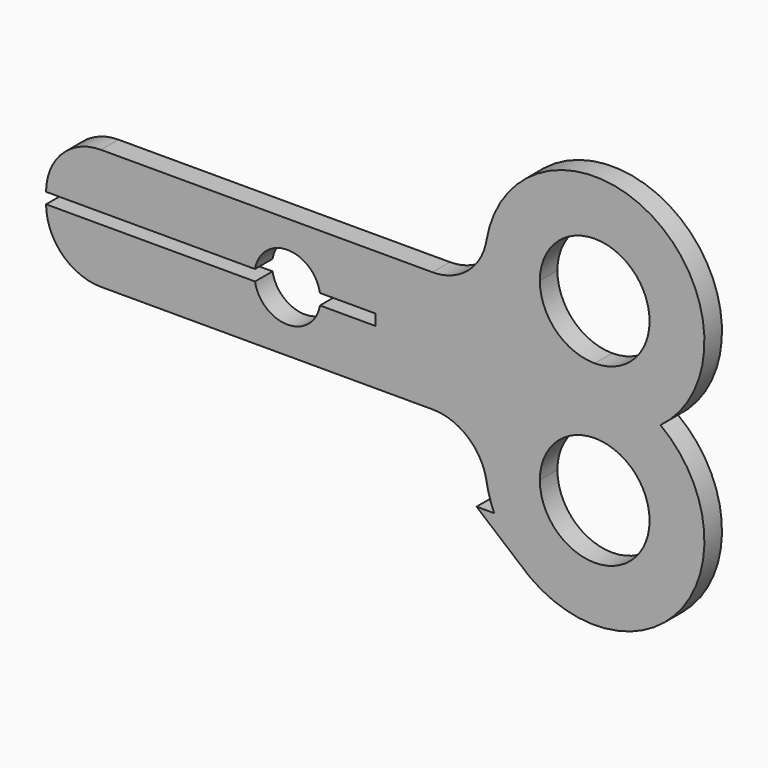
from build123d import *

# Parameters (mm, degrees)
F1_DEPTH = 2
F2_R     = 5
F4_DEPTH = 2
F6_DEPTH = 2


# Not quite as in the source:
# - a feature names something its author has since deleted; it is built from what else it names


with BuildPart() as f1:
    # F0 (on Front) → F1 (new body)
    with BuildSketch(Plane.XZ):
        with BuildLine():
            Line((0, 5.5), (0, 0))
            Line((0, 0), (40, 0))
            Line((40, 0), (40, 5.5))
            Line((40, 5.5), (25, 5.5))
            ThreePointArc((25, 5.5), (22, 2.5), (19, 5.5))
            Line((19, 5.5), (0, 5.5))
        make_face()
        with BuildLine():
            Line((40, 5.5), (40, 0))
            Line((40, 0), (40, -2.5))
            ThreePointArc((40, -2.5), (41.05572809, 1.972135955), (44, 5.5))
            Line((44, 5.5), (40, 5.5))
        make_face()
        with BuildLine():
            Line((0, 11), (0, 5.5))
            Line((0, 5.5), (19, 5.5))
            ThreePointArc((19, 5.5), (22, 8.5), (25, 5.5))
            Line((25, 5.5), (40, 5.5))
            Line((40, 5.5), (40, 11))
            Line((40, 11), (0, 11))
        make_face()
        with BuildLine():
            Line((40, 11), (40, 5.5))
            Line((40, 5.5), (44, 5.5))
            ThreePointArc((44, 5.5), (41.05572809, 9.027864045), (40, 13.5))
            Line((40, 13.5), (40, 11))
        make_face()
        with BuildLine():
            Line((45, -2.5), (40, -2.5))
            ThreePointArc((40, -2.5), (50, -12.5), (60, -2.5))
            ThreePointArc((60, -2.5), (58.94427191, 1.972135955), (56, 5.5))
            ThreePointArc((56, 5.5), (53.1622776602, 4.0131670195), (50, 3.5))
            Line((50, 3.5), (50, 2.5))
            ThreePointArc((50, 2.5), (53.5355339059, 1.0355339059), (55, -2.5))
            ThreePointArc((55, -2.5), (50, -7.5), (45, -2.5))
        make_face()
        with BuildLine():
            ThreePointArc((44, 5.5), (41.05572809, 1.972135955), (40, -2.5))
            Line((40, -2.5), (45, -2.5))
            ThreePointArc((45, -2.5), (46.4644660941, 1.0355339059), (50, 2.5))
            Line((50, 2.5), (50, 3.5))
            ThreePointArc((50, 3.5), (46.8377223398, 4.0131670195), (44, 5.5))
        make_face()
        with BuildLine():
            ThreePointArc((40, 13.5), (41.05572809, 9.027864045), (44, 5.5))
            ThreePointArc((44, 5.5), (46.8377223398, 6.9868329805), (50, 7.5))
            Line((50, 7.5), (50, 8.5))
            ThreePointArc((50, 8.5), (46.4644660941, 9.9644660941), (45, 13.5))
            Line((45, 13.5), (40, 13.5))
        make_face()
        with BuildLine():
            Line((50, 5.5), (44, 5.5))
            ThreePointArc((44, 5.5), (46.8377223398, 4.0131670195), (50, 3.5))
            Line((50, 3.5), (50, 5.5))
        make_face()
        with BuildLine():
            ThreePointArc((50, 7.5), (46.8377223398, 6.9868329805), (44, 5.5))
            Line((44, 5.5), (50, 5.5))
            Line((50, 5.5), (50, 7.5))
        make_face()
        with BuildLine():
            ThreePointArc((60, 13.5), (50, 23.5), (40, 13.5))
            Line((40, 13.5), (45, 13.5))
            ThreePointArc((45, 13.5), (50, 18.5), (55, 13.5))
            ThreePointArc((55, 13.5), (53.5355339059, 9.9644660941), (50, 8.5))
            Line((50, 8.5), (50, 7.5))
            ThreePointArc((50, 7.5), (53.1622776602, 6.9868329805), (56, 5.5))
            ThreePointArc((56, 5.5), (58.94427191, 9.027864045), (60, 13.5))
        make_face()
        with BuildLine():
            ThreePointArc((56, 5.5), (53.1622776602, 6.9868329805), (50, 7.5))
            Line((50, 7.5), (50, 5.5))
            Line((50, 5.5), (56, 5.5))
        make_face()
        with BuildLine():
            Line((50, 5.5), (50, 3.5))
            ThreePointArc((50, 3.5), (53.1622776602, 4.0131670195), (56, 5.5))
            Line((56, 5.5), (50, 5.5))
        make_face()
    extrude(amount=F1_DEPTH)

    # F2
    f2_edges = [f1.edges().sort_by_distance(p)[0] for p in [
        (40, -1, 11),
        (40, -1, 0),
        (0, -1, 11),
        (0, -1, 0),
    ]]
    fillet(f2_edges, radius=F2_R)

    # F3 (on face) → F4 (cut, through all)
    with BuildSketch(Plane.XZ.offset(2)):
        with BuildLine():
            Line((19.0419601085, 6), (0, 6))
            Line((0, 6), (0, 5))
            Line((0, 5), (19.0419601085, 5))
            ThreePointArc((19.0419601085, 5), (19, 5.5), (19.0419601085, 6))
        make_face()
        with BuildLine():
            Line((30, 6), (24.9580398915, 6))
            ThreePointArc((24.9580398915, 6), (24.9894915684, 5.7508787808), (25, 5.5))
            ThreePointArc((25, 5.5), (24.9894915684, 5.2491212192), (24.9580398915, 5))
            Line((24.9580398915, 5), (30, 5))
            Line((30, 5), (30, 6))
        make_face()
    extrude(amount=-F4_DEPTH, mode=Mode.SUBTRACT)

    # F5 (on face) → F6 (join)
    with BuildSketch(Plane.XZ.offset(2)):
        with BuildLine():
            ThreePointArc((43.1634270419, -9.7980319394), (41.8309701191, -8.2677509312), (40.8348486101, -6.5))
            Line((40.8348486101, -6.5), (39.2329856296, -6.5))
            Line((39.2329856296, -6.5), (43.1634270419, -9.7980319394))
        make_face()
    extrude(amount=-F6_DEPTH)


solid = f1.part
